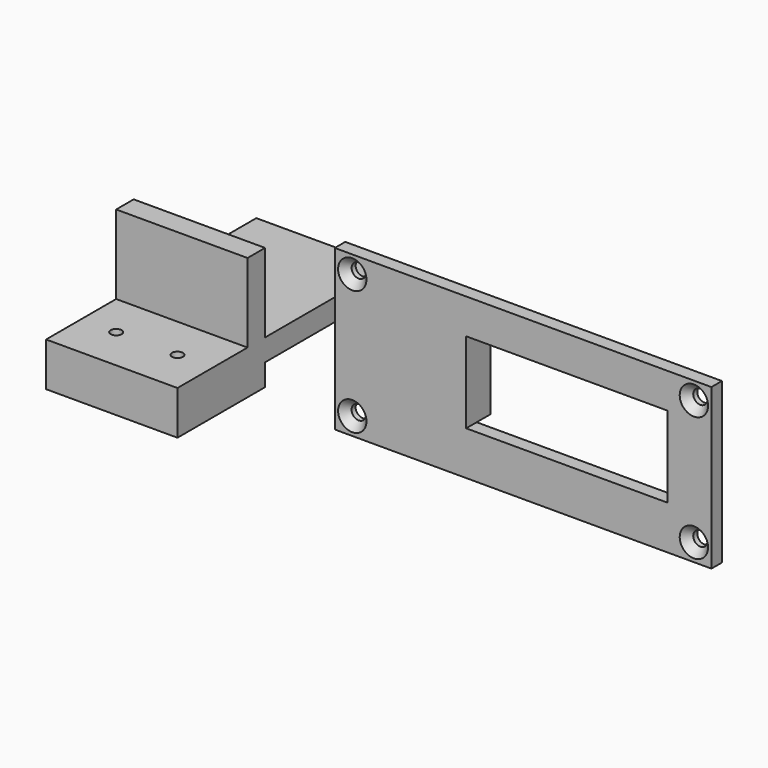
from build123d import *

# Parameters (mm, degrees)
F0_W           = 86
F0_H           = 36.5
F0_W_2         = 5
F0_H_2         = 18.5
F1_DEPTH       = 3
F2_D           = 3.2639
F2_CSINK_D     = 6.477
F2_CSINK_ANGLE = 82
F3_W           = 30
F3_H           = 18
F3_H_2         = 10
F4_DEPTH       = 5
F5_DEPTH       = 40
F5_DEPTH_BACK  = 20
F6_W           = 30
F6_H           = 30
F7_DEPTH       = 5
F9_D           = 2.5
F10_DEPTH      = 7


# Not quite as in the source:
# - a feature names something its author has since deleted; it is built from what else it names


with BuildPart() as f1:
    # F0 (on Front) → F1 (new body)
    with BuildSketch(Plane.XZ):
        with Locations((13, 8.25)):
            Rectangle(F0_W, F0_H)
        Polygon((-5, 18.5), (0, 18.5), (46, 18.5), (46, 0), (0, 0), (-5, 0), align=None, mode=Mode.SUBTRACT)
        with Locations((-2.5, 9.25)):
            Rectangle(F0_W_2, F0_H_2)
    extrude(amount=-F1_DEPTH)

    # F2 (through all)
    with Locations(Plane.XZ):
        with Locations((-26, 22.5), (52, 22.5), (52, -6), (-26, -6)):
            CounterSinkHole(F2_D / 2, F2_CSINK_D / 2, counter_sink_angle=F2_CSINK_ANGLE)

    # F0 (on Front) → F10 (join)
    with BuildSketch(Plane.XZ):
        with Locations((-2.5, 9.25)):
            Rectangle(F0_W_2, F0_H_2)
    extrude(amount=-F10_DEPTH)


with BuildPart() as f4:
    # F3 (on Front) → F4 (new body)
    with BuildSketch(Plane.XZ):
        with Locations((-64.9130126834, 9)):
            Rectangle(F3_W, F3_H)
        with Locations((-64.9130126834, -5)):
            Rectangle(F3_W, F3_H_2)
    extrude(amount=-F4_DEPTH)

    # F3 (on Front) → F5 (join, two sides)
    with BuildSketch(Plane.XZ) as f5_sk:
        with Locations((-64.9130126834, -5)):
            Rectangle(F3_W, F3_H_2)
    extrude(amount=-F5_DEPTH)
    extrude(f5_sk.sketch, amount=F5_DEPTH_BACK)

    # F6 (on face) → F7 (cut)
    with BuildSketch(Plane(origin=(0, 0, -10), x_dir=(1, 0, 0), z_dir=(0, 0, -1))):
        with Locations((-64.9130126834, -20)):
            Rectangle(F6_W, F6_H)
    extrude(amount=-F7_DEPTH, mode=Mode.SUBTRACT)

    # F9 (through all)
    with Locations(Plane.XY):
        with Locations((-71.9130126834, -10), (-57.9130126834, -10)):
            Hole(F9_D / 2)


solid = Compound([f1.part, f4.part])
